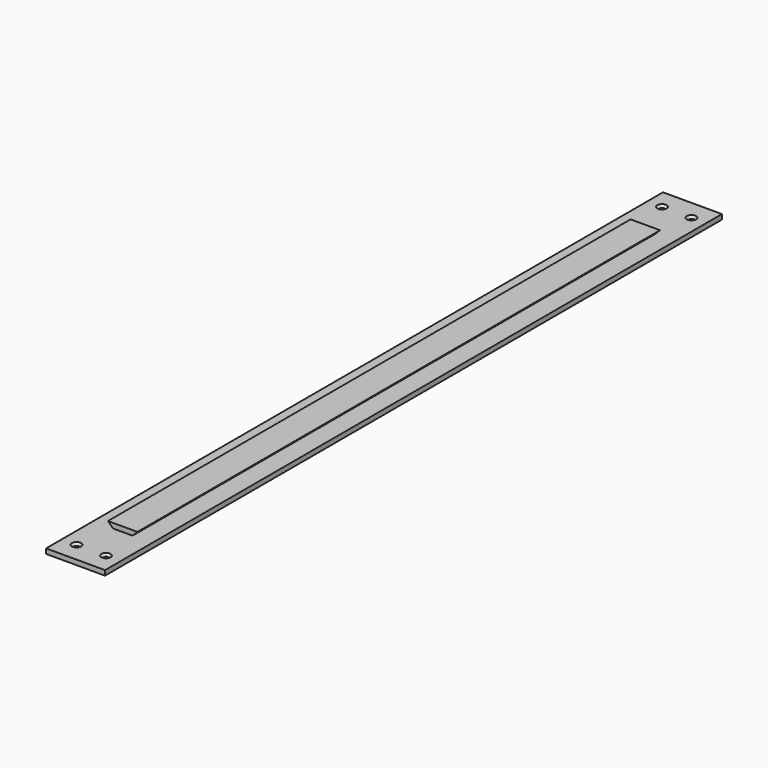
from build123d import *

# Parameters (mm, degrees)
F1_DEPTH       = 1993.9
F2_W           = 152.4
F2_H           = 152.4
F3_DEPTH       = 12.7
F5_D           = 13.49248
F5_CSINK_D     = 23.8252
F5_CSINK_ANGLE = 82


with BuildPart() as f1:
    # F0 (on Front) → F1 (new body)
    with BuildSketch(Plane.XZ):
        Polygon((0, 12.7), (0, 0), (152.4, 0), (152.4, 12.7), (101.6, 12.7), (114.3, 25.4), (38.1, 25.4), (50.8, 12.7), align=None)
    extrude(amount=F1_DEPTH)

    # F2 (on face) → F3 (cut, through all)
    with BuildSketch(Plane.XY.offset(25.4)):
        with Locations((76.2, -76.2)):
            Rectangle(F2_W, F2_H)
        with Locations((76.2, -1917.7)):
            Rectangle(F2_W, F2_H)
    extrude(amount=-F3_DEPTH, mode=Mode.SUBTRACT)

    # F5 (through all)
    with Locations(Plane.XY.offset(12.7)):
        with Locations((38.1, -50.8), (114.3, -50.8), (38.1, -1943.1), (114.3, -1943.1)):
            CounterSinkHole(F5_D / 2, F5_CSINK_D / 2, counter_sink_angle=F5_CSINK_ANGLE)


solid = f1.part
